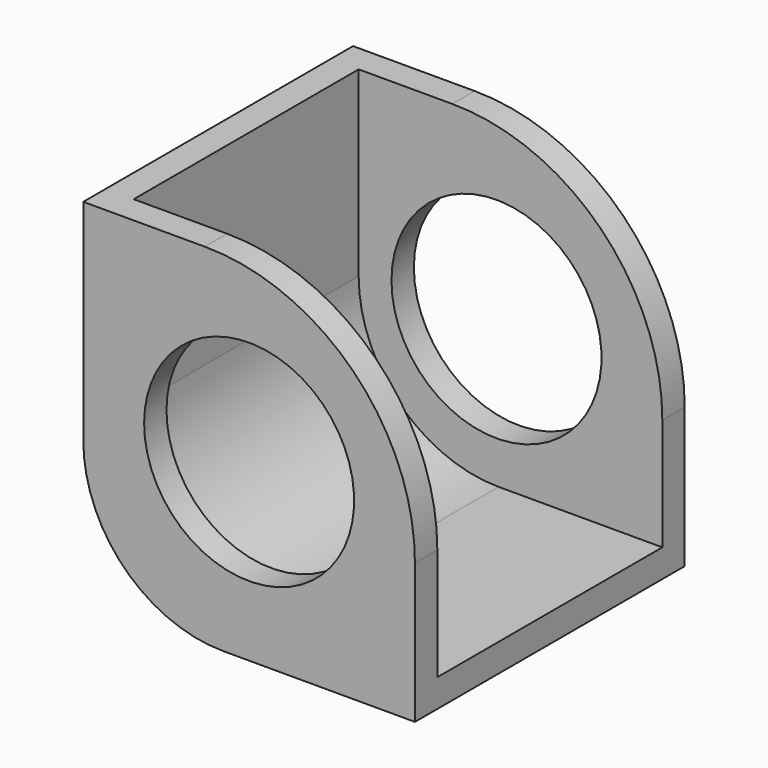
from build123d import *

# Parameters (mm, degrees)
F0_W     = 60.1664371789
F0_H     = 61.1762590706
F1_DEPTH = 63.5
F2_T     = -5.08
F3_R     = 19.05
F4_DEPTH = 61.1762590706
F5_R     = 38.1
F7_R     = 25.4


# Not quite as in the source:
# - a feature of the source that left no trace in its solid (it failed there, or was rolled back) is left out


with BuildPart() as f1:
    # F0 (on Top) → F1 (new body)
    with BuildSketch(Plane.XY):
        Rectangle(F0_W, F0_H)
    extrude(amount=F1_DEPTH)

    # F2
    f2_openings = [f1.faces().sort_by_distance(p)[0] for p in [
        (30.083219, 0, 31.75),
        (0, 0, 63.5),
    ]]
    offset(amount=F2_T, openings=f2_openings)

    # F3 (on face) → F4 (cut, through all)
    with BuildSketch(Plane(origin=(0, 30.5881295353, 0), x_dir=(-1, 0, 0), z_dir=(0, 1, 0))):
        with Locations((0, 31.75)):
            Circle(F3_R)
    extrude(amount=-F4_DEPTH, mode=Mode.SUBTRACT)

    # F5
    f5_edges = [f1.edges().sort_by_distance(p)[0] for p in [
        (30.083219, -28.04813, 63.5),
        (30.083219, 28.04813, 63.5),
    ]]
    fillet(f5_edges, radius=F5_R)

    # F7
    f7_edges = [f1.edges().sort_by_distance(p)[0] for p in [
        (-30.083219, 0, 0),
        (-25.003219, 0, 5.08),
    ]]
    fillet(f7_edges, radius=F7_R)


solid = f1.part
